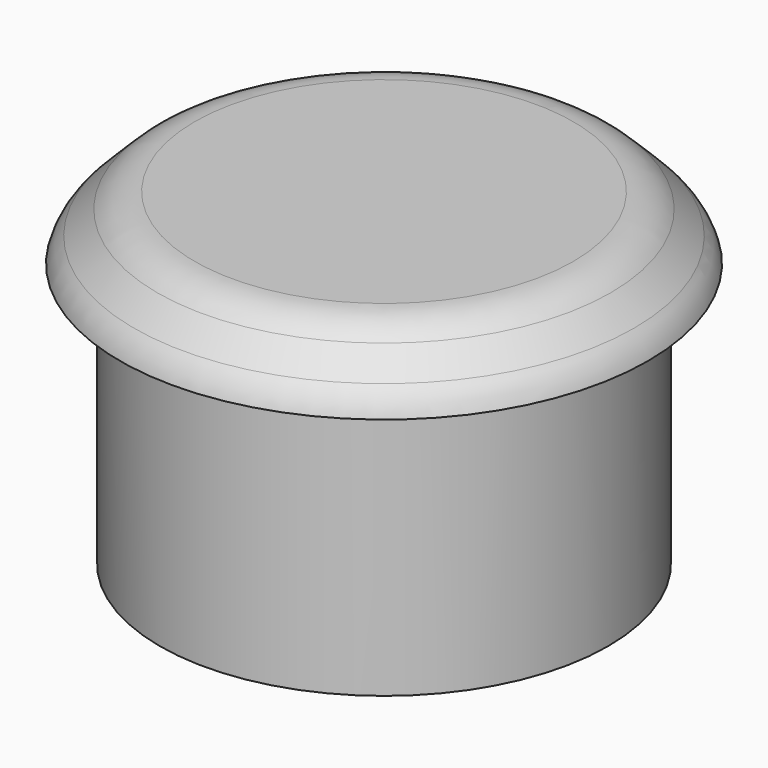
from build123d import *

# Parameters (mm, degrees)
F0_R     = 25
F1_DEPTH = 6
F2_R     = 21.4280280098
F3_DEPTH = 3
F4_SIZE  = 5
F6_R     = 21.8410066176
F7_DEPTH = 4
F8_R     = 21.2290439381
F9_DEPTH = 25


# Not quite as in the source:
# - a fillet or chamfer that OpenCascade refuses, or shapes differently, is made with other operations: its cross-section is extruded or revolved along the edge and cut away or added


with BuildPart() as f1:
    # F0 (on Top) → F1 (new body)
    with BuildSketch(Plane.XY):
        Circle(F0_R)
    extrude(amount=F1_DEPTH)

    # F2 (on face) → F3 (join)
    with BuildSketch(Plane.XY.offset(6)):
        Circle(F2_R)
    extrude(amount=-F3_DEPTH)

    # F4
    f4_edges = [f1.edges().sort_by_distance(p)[0] for p in [
        (-25, 0, 6),
    ]]
    chamfer(f4_edges, length=F4_SIZE)

    # F5: fillet of radius 5 on 3 edges, made by hand

    # F5_s1 → F5_t2 (revolve, cut)
    with BuildSketch(Plane.XZ):
        with BuildLine():
            ThreePointArc((25, 0), (24.5002551285, 1.2451619378), (23.687395822, 2.312604178))
            Line((23.687395822, 2.312604178), (25, 1))
            Line((25, 1), (25, 0))
        make_face()
    revolve(axis=Axis((0, 0, 1), (0, 0, 1)), mode=Mode.SUBTRACT)

    # F5_s3 → F5_t4 (revolve, cut)
    with BuildSketch(Plane.XZ):
        with BuildLine():
            ThreePointArc((21.4644660941, 4.5355339059), (19.84234935, 5.6193976626), (17.9289321881, 6))
            Line((17.9289321881, 6), (20, 6))
            Line((20, 6), (21.4644660941, 4.5355339059))
        make_face()
    revolve(axis=Axis((0, 0, 6), (0, 0, 1)), mode=Mode.SUBTRACT)

    # F6 (on face) → F7 (join)
    with BuildSketch(Plane(origin=(0, 0, 0), x_dir=(1, 0, 0), z_dir=(0, 0, -1))):
        Circle(F6_R)
    extrude(amount=-F7_DEPTH)

    # F8 (on face) → F9 (join)
    with BuildSketch(Plane(origin=(0, 0, 0), x_dir=(1, 0, 0), z_dir=(0, 0, -1))):
        Circle(F8_R)
    extrude(amount=F9_DEPTH)


solid = f1.part
